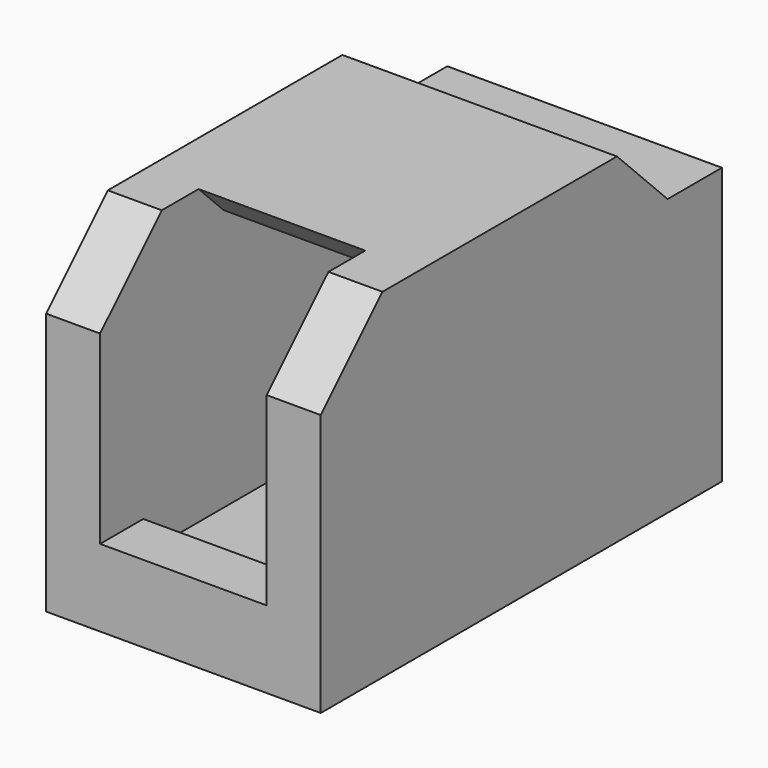
from build123d import *

# Parameters (mm, degrees)
F1_DEPTH     = 3
F0_W         = 3.4999997824
F0_H         = 12.75
F2_DEPTH     = 22
F0_W_2       = 10.8
F0_H_2       = 3.4999997824
F3_DEPTH     = 5
F4_SIZE      = 5
F5_DEPTH     = 17.9
F6_T4_DEPTH  = 29.2168296621
F6_T9_DEPTH  = 29.2168296621
F7_W         = 3.4999997824
F7_H         = 4.4000236183
F8_DEPTH     = 8.1
F9_W         = 3.4999997824
F9_H         = 5.7981096033
F9_H_2       = 0.0001660025
F9_W_2       = 14.2999671862
F10_DEPTH    = 1.59
F11_DEPTH    = 5
F13_DEPTH    = 2.02
F14_T4_DEPTH = 36.5168298797


# Not quite as in the source:
# - a fillet or chamfer that OpenCascade refuses, or shapes differently, is made with other operations: its cross-section is extruded or revolved along the edge and cut away or added
# - ends of sketch curves that miss each other by under 0.0002 mm in the source are joined


with BuildPart() as f1:
    # F0 (on Top) → F1 (new body)
    with BuildSketch(Plane.XY):
        Polygon((5.4, 0), (5.4, 12.75), (-5.4, 12.75), (-5.4, 0), (-5.4, -12.75), (5.4, -12.75), align=None)
    extrude(amount=F1_DEPTH)

    # F0 (on Top) → F2 (join)
    with BuildSketch(Plane.XY):
        with Locations((-7.1499998912, 6.375)):
            Rectangle(F0_W, F0_H)
        with Locations((7.1499998912, 6.375)):
            Rectangle(F0_W, F0_H)
        Polygon((-5.4, -12.75), (-5.4, 0), (-8.8999997824, 0), (-8.8999997824, -16.2499997824), (-5.4, -16.2499997824), align=None)
        Polygon((8.8999997824, 0), (5.4, 0), (5.4, -12.75), (5.4, -16.2499997824), (8.8999997824, -16.2499997824), align=None)
    extrude(amount=F2_DEPTH)

    # F0 (on Top) → F3 (join)
    with BuildSketch(Plane.XY):
        with Locations((0, 14.4999998912)):
            Rectangle(F0_W_2, F0_H_2)
        with Locations((-7.1499998912, 14.4999998912)):
            Rectangle(F0_W, F0_H_2)
        with Locations((7.1499998912, 14.4999998912)):
            Rectangle(F0_W, F0_H_2)
    extrude(amount=F3_DEPTH)

    # F4
    f4_edges = [f1.edges().sort_by_distance(p)[0] for p in [
        (-7.15, -16.25, 22),
        (7.15, -16.25, 22),
    ]]
    chamfer(f4_edges, length=F4_SIZE)

    # F0 (on Top) → F5 (join)
    with BuildSketch(Plane.XY):
        with Locations((-7.1499998912, 14.4999998912)):
            Rectangle(F0_W, F0_H_2)
        with Locations((7.1499998912, 14.4999998912)):
            Rectangle(F0_W, F0_H_2)
    extrude(amount=F5_DEPTH)

    # F6: chamfer of 5 on 2 edges, made by hand


with BuildPart() as f6_tool2:
    # F6_s3 → F6_t4 (new body)
    with BuildSketch(Plane.YZ.offset(21.7584147223)):
        Polygon((7.75, 22), (12.75, 17), (12.75, 22), align=None)
    extrude(amount=-F6_T4_DEPTH)

    split(bisect_by=Plane.XY.offset(17.9), keep=Keep.TOP)


with BuildPart() as f1_1:
    add(f1.part)

    # F6_t1: cut F6_tool2
    add(f6_tool2.part, mode=Mode.SUBTRACT)


with BuildPart() as f6_tool7:
    # F6_s8 → F6_t9 (new body)
    with BuildSketch(Plane.YZ.offset(7.4584149398)):
        Polygon((12.75, 17), (7.75, 22), (12.75, 22), align=None)
    extrude(amount=-F6_T9_DEPTH)

    split(bisect_by=Plane.XY.offset(17.9), keep=Keep.TOP)


with BuildPart() as f1_2:
    add(f1_1.part)

    # F6_t6: cut F6_tool7
    add(f6_tool7.part, mode=Mode.SUBTRACT)

    # F7 (on face) → F8 (join)
    with BuildSketch(Plane.XY.offset(17.9)):
        with Locations((7.1499998912, 14.0500118092)):
            Rectangle(F7_W, F7_H)
        Polygon((-8.9000016451, 11.85), (5.4, 11.85), (5.4, 16.2499997824), (-8.9000016451, 16.2500236183), align=None)
    extrude(amount=-F8_DEPTH)

    # F9 (on face) → F10 (join)
    with BuildSketch(Plane(origin=(0, 14.875, 14.875), x_dir=(-1, 0, 0), z_dir=(0, 0.7071067812, 0.7071067812))):
        with Locations((-7.1499998912, 7.1772168303)):
            Rectangle(F9_W, F9_H)
        with Locations((-7.1499998912, 4.2780790274)):
            Rectangle(F9_W, F9_H_2)
        with Locations((1.7499835931, 7.1772168303)):
            Rectangle(F9_W_2, F9_H)
    extrude(amount=-F10_DEPTH)

    # F0 (on Top) → F11 (join)
    with BuildSketch(Plane.XY):
        with Locations((0, -14.4999998912)):
            Rectangle(F0_W_2, F0_H_2)
    extrude(amount=F11_DEPTH)

    # F12 (on face) → F13 (join)
    with BuildSketch(Plane.XY.offset(22)):
        Polygon((5.4, -11.2499997824), (5.4, 7.75), (-8.8998991996, 7.75), (-8.8998991996, -11.2499557436), align=None)
    extrude(amount=-F13_DEPTH)

    # F14: chamfer of 5 on 1 edges, made by hand


with BuildPart() as f14_tool2:
    # F14_s3 → F14_t4 (new body)
    with BuildSketch(Plane(origin=(-18.2583802936, 5.62297e-05, 0), x_dir=(0, 0, 1), z_dir=(1, -3.0797e-06, 0))):
        Polygon((19.98, 6.2499831522), (24.98, 11.2499831522), (19.98, 11.2499831522), align=None)
    extrude(amount=F14_T4_DEPTH)

    split(bisect_by=Plane.YZ.offset(5.4), keep=Keep.BOTTOM)

    split(bisect_by=Plane.YZ.offset(-5.4), keep=Keep.TOP)


with BuildPart() as f1_3:
    add(f1_2.part)

    # F14_t1: cut F14_tool2
    add(f14_tool2.part, mode=Mode.SUBTRACT)


solid = f1_3.part
